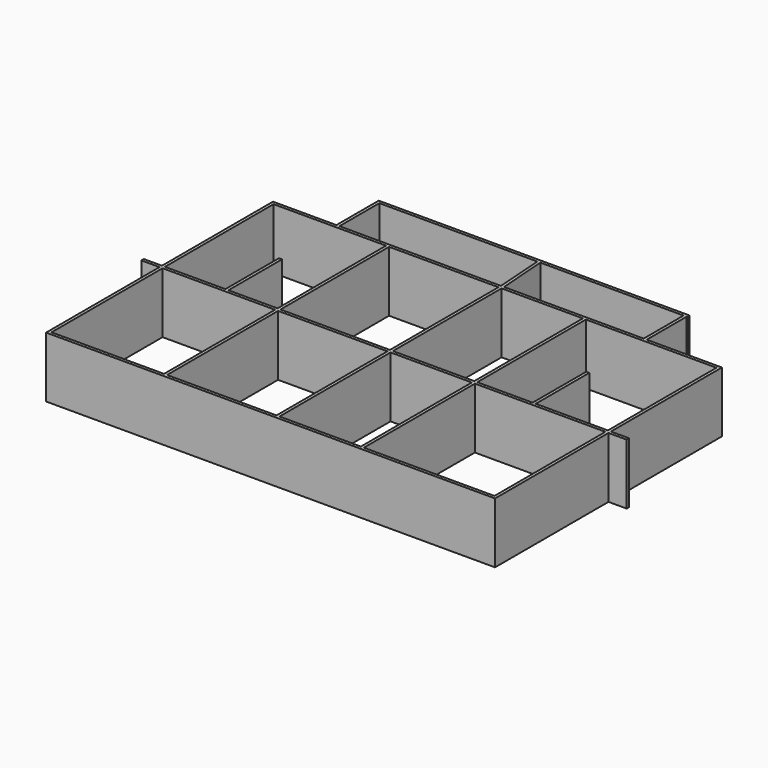
from build123d import *

# Parameters (mm, degrees)
F0_W     = 37.0614326914
F0_H     = 45.7304640924
F0_W_2   = 26.8021334539
F0_W_3   = 43.0278818478
F0_H_2   = 44.7304640924
F1_DEPTH = 20


with BuildPart() as f1:
    # F0 (on Top) → F1 (new body)
    with BuildSketch(Plane.XY):
        Polygon((73.9764403422, 1), (73.9764403422, 46.7304640924), (49.1905527413, 46.7304640924), (49.1905527413, 63.1642210121), (49.4113042951, 63.1642210121), (49.4113042951, 64.1642210121), (-53.0780255795, 64.1642210121), (-53.0780255795, 63.1642210121), (-53.0780255795, 46.7304640924), (-73.9764403422, 46.7304640924), (-73.9764403422, 1), (-79.9764403422, 1), (-79.9764403422, 0), (-73.9764403422, 0), (-73.9764403422, -46.7304640924), (73.9764403422, -46.7304640924), (73.9764403422, 0), (79.9764403422, 0), (79.9764403422, 1), align=None)
        with Locations((-54.4457239965, -22.8652320462)):
            Rectangle(F0_W, F0_H, mode=Mode.SUBTRACT)
        Polygon((-34.9150076509, 45.7304640924), (1.1464250405, 45.7304640924), (1.1464250405, 1), (1.1464250405, 0), (1.1464250405, -45.7304640924), (-34.9150076509, -45.7304640924), (-34.9150076509, 0), (-34.9150076509, 1), align=None, mode=Mode.SUBTRACT)
        with Locations((15.5474917675, -22.8652320462)):
            Rectangle(F0_W_2, F0_H, mode=Mode.SUBTRACT)
        with Locations((51.4624994183, -22.8652320462)):
            Rectangle(F0_W_3, F0_H, mode=Mode.SUBTRACT)
        Polygon((-72.9764403422, 1), (-72.9764403422, 45.7304640924), (-35.9150076509, 45.7304640924), (-35.9150076509, 1), (-52.0780255795, 1), (-52.0780255795, 23.0720378458), (-53.0780255795, 23.0720378458), (-53.0780255795, 1), align=None, mode=Mode.SUBTRACT)
        Polygon((-52.0780255795, 63.1642210121), (0, 63.1642210121), (1.1464250405, 46.7304640924), (-52.0780255795, 46.7304640924), align=None, mode=Mode.SUBTRACT)
        with Locations((15.5474917675, 23.3652320462)):
            Rectangle(F0_W_2, F0_H_2, mode=Mode.SUBTRACT)
        Polygon((29.9485584944, 1), (29.9485584944, 45.7304640924), (72.9764403422, 45.7304640924), (72.9764403422, 1), (49.1905527413, 1), (49.1905527413, 23.0720378458), (48.1905527413, 23.0720378458), (48.1905527413, 1), align=None, mode=Mode.SUBTRACT)
        Polygon((1, 63.1642210121), (48.1905527413, 63.1642210121), (48.1905527413, 46.7304640924), (2.1464250405, 46.7304640924), align=None, mode=Mode.SUBTRACT)
        Polygon((1.1464250405, 0), (1.1464250405, 1), (-34.9150076509, 1), (-34.9150076509, 0), (0, 0), align=None)
    extrude(amount=F1_DEPTH)


solid = f1.part
